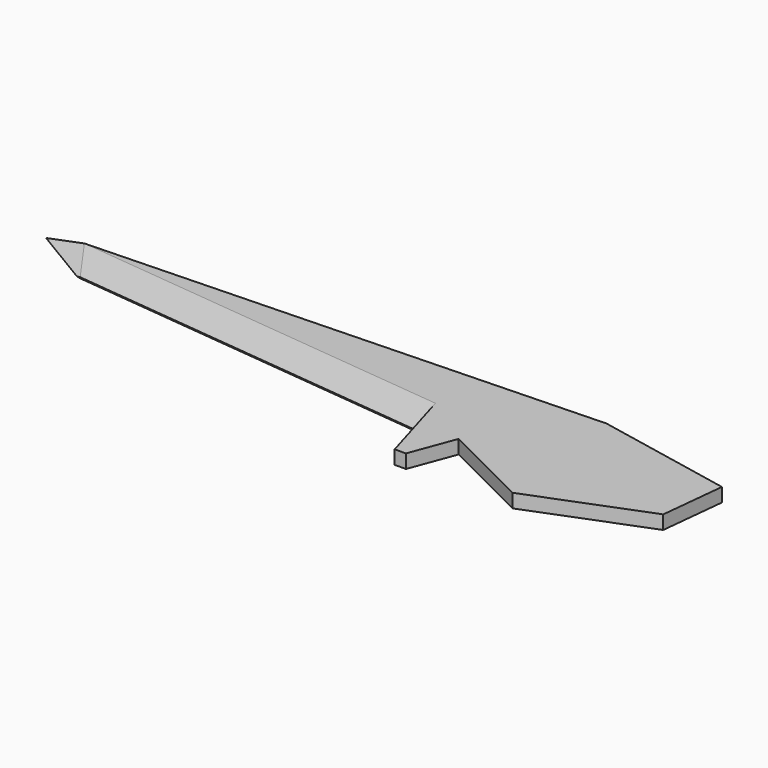
from build123d import *

# Parameters (mm, degrees)
F1_DEPTH    = 2
F2_SIZE2    = 1.85
F2_SIZE     = 10
F2_2_SIZE2  = 1.85
F2_2_SIZE   = 10
F3_T1_DEPTH = 63.0781913019
F3_T3_DEPTH = 63.0781913019


# Not quite as in the source:
# - a fillet or chamfer that OpenCascade refuses, or shapes differently, is made with other operations: its cross-section is extruded or revolved along the edge and cut away or added


with BuildPart() as f1:
    # F0 (on Top) → F1 (new body, symmetric)
    with BuildSketch(Plane.XY):
        Polygon((-78.3224657339, 21.585099696), (-72.0955598013, 12.517264094), (48.031361701, 0), (51.9027564591, -13.106621107), (55.166546928, -13.106621107), (60.0622307678, 0), (86.172547065, -13.106621107), (119.6195638295, 0), (121.5894543095, 18.9048403295), (81.5894543095, 26.893378893), align=None)
    extrude(amount=F1_DEPTH, both=True)

    # F2
    f2_edges = [f1.edges().sort_by_distance(p)[0] for p in [
        (-12.032099, 6.258632, 2),
    ]]
    f2_side = f1.faces().sort_by_distance((40.734375, 11.652616, 2))[0]
    chamfer(f2_edges, length=F2_SIZE, length2=F2_SIZE2, reference=f2_side)

    # F2#2
    f2_2_edges = [f1.edges().sort_by_distance(p)[0] for p in [
        (-12.032099, 6.258632, -2),
    ]]
    f2_2_side = f1.faces().sort_by_distance((40.734375, 11.652616, -2))[0]
    chamfer(f2_2_edges, length=F2_2_SIZE, length2=F2_2_SIZE2, reference=f2_2_side)

    # F3: chamfer of 1.85 x 10 on 2 edges, made by hand

    # F3_s2 → F3_t1 (cut)
    with BuildSketch(Plane(origin=(-49.185702612, 71.6259198522, -12.2363892176), x_dir=(0.8243486911, 0.5660823575, 0), z_dir=(0.5605509501, -0.8162936645, 0.1394535249))):
        Polygon((-52.3460779882, 8.8318101599), (-42.4159004982, 5.802159781), (-52.3460779882, 6.9818101599), align=None)
    extrude(amount=F3_T1_DEPTH, mode=Mode.SUBTRACT)

    # F3_s4 → F3_t3 (cut)
    with BuildSketch(Plane(origin=(-49.185702612, 71.6259198522, 12.2363892176), x_dir=(0.8243486911, 0.5660823575, 0), z_dir=(0.5605509501, -0.8162936645, -0.1394535249))):
        Polygon((-52.3460779882, -8.8318101599), (-42.4159004982, -5.802159781), (-52.3460779882, -6.9818101599), align=None)
    extrude(amount=F3_T3_DEPTH, mode=Mode.SUBTRACT)


solid = f1.part
